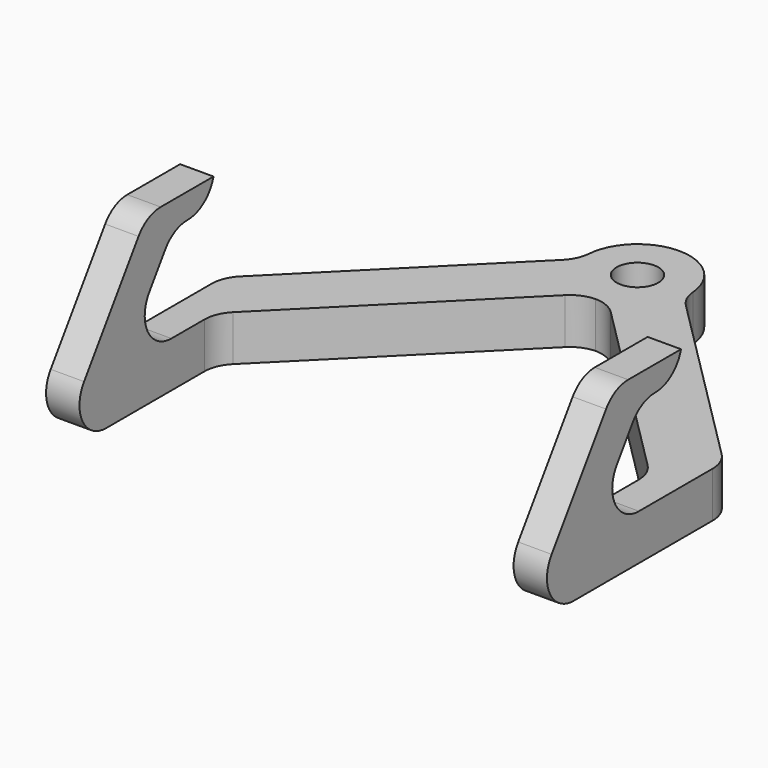
from build123d import *

# Parameters (mm, degrees)
F0_W          = 76.2
F0_H          = 76.2
F1_DEPTH      = 25.4
F3_DEPTH      = 38.1
F5_DEPTH      = 25.401
F6_R          = 3.175
F7_DEPTH      = 6.9583890807
F8_DEPTH      = 25.4
F9_R          = 5.08
F10_T1_DEPTH  = 6.9583890807
F10_T3_DEPTH  = 5.08
F10_T5_DEPTH  = 5.08
F10_T7_DEPTH  = 53.0515000437
F10_T9_DEPTH  = 53.0515000437
F10_T11_DEPTH = 18.5288185571
F10_T13_DEPTH = 18.5288185571
F10_T15_DEPTH = 29.6734442484
F10_T17_DEPTH = 29.6734442484


# Not quite as in the source:
# - a fillet or chamfer that OpenCascade refuses, or shapes differently, is made with other operations: its cross-section is extruded or revolved along the edge and cut away or added


with BuildPart() as f1:
    # F0 (on Top) → F1 (new body)
    with BuildSketch(Plane.XY):
        Rectangle(F0_W, F0_H)
    extrude(amount=F1_DEPTH)

    # F2 (on Right) → F3 (cut, symmetric)
    with BuildSketch(Plane.YZ):
        Polygon((-38.1, 25.4), (-38.1, 0), (-20.8386592567, 25.4), align=None)
        Polygon((38.1, 6.9583890807), (38.1, 25.4), (-8.0999151611, 25.4), (-8.0999151611, 21.59), (-15.7503205431, 21.59), (-25.6936757282, 6.9583890807), align=None)
    extrude(amount=F3_DEPTH, both=True, mode=Mode.SUBTRACT)

    # F4 (on Top) → F5 (cut, through all)
    with BuildSketch(Plane.XY):
        Polygon((0, 38.1), (38.1, 0), (38.1, 38.1), align=None)
        Polygon((-38.1, 0), (0, 38.1), (-38.1, 38.1), align=None)
        Polygon((-33.02, -7.7263666582), (-33.02, -38.1), (33.02, -38.1), (33.02, -7.7263666582), (0, 25.2936333418), align=None)
    extrude(amount=F5_DEPTH, mode=Mode.SUBTRACT)

    # F6 (on face) → F7 (join, through all)
    with BuildSketch(Plane.XY):
        with BuildLine():
            ThreePointArc((-4.005332333, 38.1), (-3.950416488, 24.3625454142), (7.9375, 31.2471743673))
            ThreePointArc((7.9375, 31.2471743673), (6.8846289531, 35.1975908553), (4.005332333, 38.1))
            Line((4.005332333, 38.1), (-4.005332333, 38.1))
        make_face()
        with Locations((0, 31.2471743673)):
            Circle(F6_R, mode=Mode.SUBTRACT)
        with BuildLine():
            Line((-4.005332333, 38.1), (4.005332333, 38.1))
            ThreePointArc((4.005332333, 38.1), (0, 39.1846743673), (-4.005332333, 38.1))
        make_face()
    extrude(amount=F7_DEPTH)

    # F6 (on face) → F8 (cut)
    with BuildSketch(Plane.XY):
        with Locations((0, 31.2471743673)):
            Circle(F6_R)
    extrude(amount=F8_DEPTH, mode=Mode.SUBTRACT)

    # F9
    f9_edges = [f1.edges().sort_by_distance(p)[0] for p in [
        (-35.56, -25.693676, 6.958389),
        (-33.02, -7.726367, 3.479195),
        (-38.1, 0, 3.479195),
        (33.02, -7.726367, 3.479195),
        (38.1, 0, 3.479195),
        (35.56, -25.693676, 6.958389),
    ]]
    fillet(f9_edges, radius=F9_R)

    # F10: fillet of radius 5.08 on 12 edges, made by hand

    # F10_s2 → F10_t1 (join)
    with BuildSketch(Plane.XY):
        with BuildLine():
            ThreePointArc((7.910990874, 31.8953484504), (8.3640781537, 30.1759845193), (9.3819225849, 28.7180774151))
            Line((9.3819225849, 28.7180774151), (7.8718203721, 30.2281796279))
            ThreePointArc((7.8718203721, 30.2281796279), (7.9353100556, 31.0607324947), (7.910990874, 31.8953484504))
        make_face()
        with BuildLine():
            ThreePointArc((-9.3819225849, 28.7180774151), (-8.3640781537, 30.1759845193), (-7.910990874, 31.8953484504))
            ThreePointArc((-7.910990874, 31.8953484504), (-7.9353100556, 31.0607324947), (-7.8718203721, 30.2281796279))
            Line((-7.8718203721, 30.2281796279), (-9.3819225849, 28.7180774151))
        make_face()
        with BuildLine():
            ThreePointArc((-3.4712959528, 21.8223373889), (-1.8449823337, 22.9144717277), (0.0736624973, 23.3100161802))
            ThreePointArc((0.0736624973, 23.3100161802), (-0.8598619388, 23.3563858328), (-1.7814634495, 23.5121698923))
            Line((-1.7814634495, 23.5121698923), (-3.4712959528, 21.8223373889))
        make_face()
        with BuildLine():
            ThreePointArc((-0.0736624973, 23.3100161802), (1.8449823337, 22.9144717277), (3.4712959528, 21.8223373889))
            Line((3.4712959528, 21.8223373889), (1.7814634495, 23.5121698923))
            ThreePointArc((1.7814634495, 23.5121698923), (0.8598619388, 23.3563858328), (-0.0736624973, 23.3100161802))
        make_face()
    extrude(amount=F10_T1_DEPTH)

    # F10_s4 → F10_t3 (join)
    with BuildSketch(Plane.YZ.offset(33.02)):
        with BuildLine():
            ThreePointArc((-17.2621631711, 19.3653290824), (-15.4376693933, 20.9995139903), (-13.0605568317, 21.59))
            Line((-13.0605568317, 21.59), (-15.7503205431, 21.59))
            Line((-15.7503205431, 21.59), (-17.2621631711, 19.3653290824))
        make_face()
    extrude(amount=F10_T3_DEPTH)

    # F10_s6 → F10_t5 (join)
    with BuildSketch(Plane.YZ.offset(-38.1)):
        with BuildLine():
            ThreePointArc((-17.2621631711, 19.3653290824), (-15.4376693933, 20.9995139903), (-13.0605568317, 21.59))
            Line((-13.0605568317, 21.59), (-15.7503205431, 21.59))
            Line((-15.7503205431, 21.59), (-17.2621631711, 19.3653290824))
        make_face()
    extrude(amount=F10_T5_DEPTH)

    # F10_s8 → F10_t7 (cut)
    with BuildSketch(Plane.YZ.offset(9.0342499781)):
        with BuildLine():
            ThreePointArc((-28.5056999913, 0), (-32.9952139816, 2.7028874384), (-32.7073063306, 7.9353290824))
            Line((-32.7073063306, 7.9353290824), (-38.1, 0))
            Line((-38.1, 0), (-28.5056999913, 0))
        make_face()
    extrude(amount=F10_T7_DEPTH, mode=Mode.SUBTRACT)

    # F10_s10 → F10_t9 (cut)
    with BuildSketch(Plane.YZ.offset(-62.0857500219)):
        with BuildLine():
            ThreePointArc((-28.5056999913, 0), (-32.9952139816, 2.7028874384), (-32.7073063306, 7.9353290824))
            Line((-32.7073063306, 7.9353290824), (-38.1, 0))
            Line((-38.1, 0), (-28.5056999913, 0))
        make_face()
    extrude(amount=F10_T9_DEPTH, mode=Mode.SUBTRACT)

    # F10_s12 → F10_t11 (cut)
    with BuildSketch(Plane.YZ.offset(26.2955907214)):
        with BuildLine():
            ThreePointArc((-22.3505018847, 23.1753290824), (-20.5260081069, 24.8095139903), (-18.1488955453, 25.4))
            Line((-18.1488955453, 25.4), (-20.8386592567, 25.4))
            Line((-20.8386592567, 25.4), (-22.3505018847, 23.1753290824))
        make_face()
    extrude(amount=F10_T11_DEPTH, mode=Mode.SUBTRACT)

    # F10_s14 → F10_t13 (cut)
    with BuildSketch(Plane.YZ.offset(-44.8244092786)):
        with BuildLine():
            ThreePointArc((-22.3505018847, 23.1753290824), (-20.5260081069, 24.8095139903), (-18.1488955453, 25.4))
            Line((-18.1488955453, 25.4), (-20.8386592567, 25.4))
            Line((-20.8386592567, 25.4), (-22.3505018847, 23.1753290824))
        make_face()
    extrude(amount=F10_T13_DEPTH, mode=Mode.SUBTRACT)

    # F10_s16 → F10_t15 (cut)
    with BuildSketch(Plane.YZ.offset(20.7232778758)):
        with BuildLine():
            ThreePointArc((-8.0999151611, 25.4), (-9.9077520374, 22.6539073716), (-13.0186040108, 21.59))
            Line((-13.0186040108, 21.59), (-8.0999151611, 21.59))
            Line((-8.0999151611, 21.59), (-8.0999151611, 25.4))
        make_face()
    extrude(amount=F10_T15_DEPTH, mode=Mode.SUBTRACT)

    # F10_s18 → F10_t17 (cut)
    with BuildSketch(Plane.YZ.offset(-50.3967221242)):
        with BuildLine():
            ThreePointArc((-8.0999151611, 25.4), (-9.9077520374, 22.6539073716), (-13.0186040108, 21.59))
            Line((-13.0186040108, 21.59), (-8.0999151611, 21.59))
            Line((-8.0999151611, 21.59), (-8.0999151611, 25.4))
        make_face()
    extrude(amount=F10_T17_DEPTH, mode=Mode.SUBTRACT)


solid = f1.part
